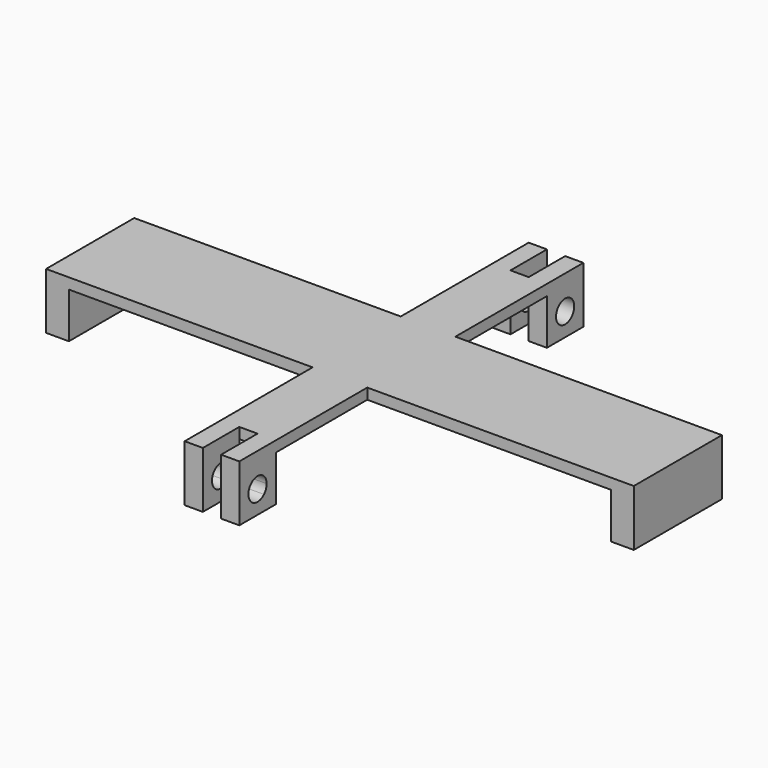
from build123d import *

# Parameters (mm, degrees)
F1_DEPTH = 3
F2_W     = 5.08
F2_H     = 12.7
F2_W_2   = 6.35
F2_H_2   = 30.7130107253
F3_DEPTH = 12.7
F4_R     = 3.175
F5_DEPTH = 25.4


with BuildPart() as f1:
    # F0 (on Top) → F1 (new body)
    with BuildSketch(Plane.XY):
        Polygon((-2.54, 59.944), (-7.62, 59.944), (-7.62, 15.3565053627), (-81.915, 15.3565053627), (-81.915, -15.3565053627), (-7.62, -15.3565053627), (-7.62, -59.944), (-2.54, -59.944), (-2.54, -53.594), (-2.54, -47.244), (2.54, -47.244), (2.54, -59.944), (2.8766005316, -59.944), (6.35, -59.944), (7.62, -59.944), (7.62, -15.3565053627), (81.915, -15.3565053627), (81.915, 15.3565053627), (7.62, 15.3565053627), (7.62, 59.944), (6.35, 59.944), (2.8766005316, 59.944), (2.54, 59.944), (2.54, 47.244), (-2.54, 47.244), (-2.54, 53.594), align=None)
    extrude(amount=F1_DEPTH)

    # F2 (on face) → F3 (join)
    with BuildSketch(Plane(origin=(0, 0, 0), x_dir=(1, 0, 0), z_dir=(0, 0, -1))):
        with Locations((-5.08, 53.594)):
            Rectangle(F2_W, F2_H)
        with Locations((5.08, 53.594)):
            Rectangle(F2_W, F2_H)
        with Locations((78.74, 0)):
            Rectangle(F2_W_2, F2_H_2)
        with Locations((5.08, -53.594)):
            Rectangle(F2_W, F2_H)
        with Locations((-5.08, -53.594)):
            Rectangle(F2_W, F2_H)
        with Locations((-78.74, 0)):
            Rectangle(F2_W_2, F2_H_2)
    extrude(amount=F3_DEPTH)

    # F4 (on face) → F5 (cut)
    with BuildSketch(Plane.YZ.offset(7.62)):
        with Locations((53.594, -6.35)):
            Circle(F4_R)
        with BuildLine():
            Line((-55.8390640303, -4.1049359697), (-51.3489359697, -8.5950640303))
            ThreePointArc((-51.3489359697, -8.5950640303), (-50.6606824843, -7.5650198978), (-50.419, -6.35))
            ThreePointArc((-50.419, -6.35), (-52.3789801022, -3.4166824843), (-55.8390640303, -4.1049359697))
        make_face()
        with BuildLine():
            ThreePointArc((-55.8390640303, -4.1049359697), (-55.8390640303, -8.5950640303), (-51.3489359697, -8.5950640303))
            Line((-51.3489359697, -8.5950640303), (-55.8390640303, -4.1049359697))
        make_face()
    extrude(amount=-F5_DEPTH, mode=Mode.SUBTRACT)


solid = f1.part
